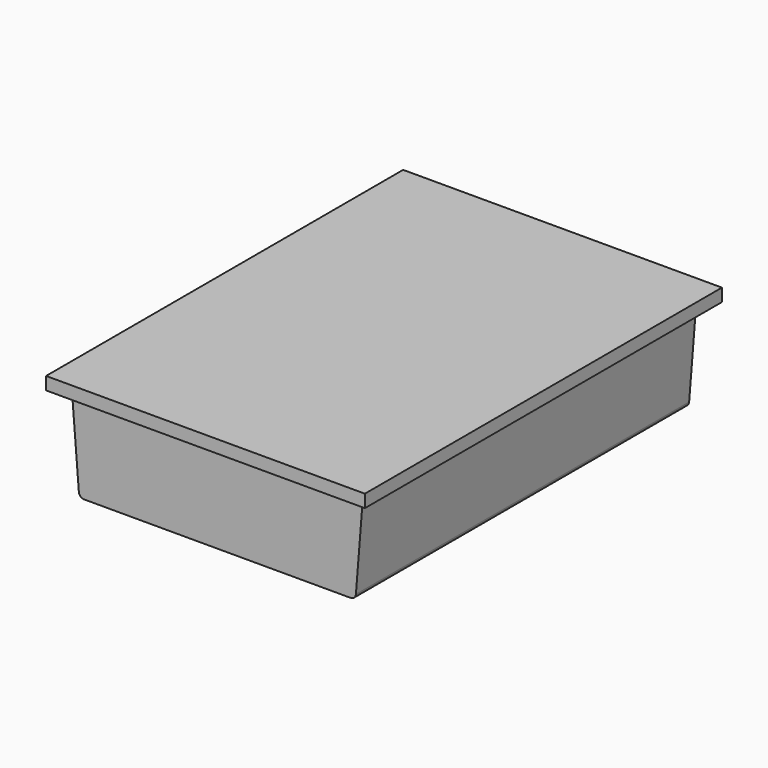
from build123d import *

# Parameters (mm, degrees)
F1_DEPTH = 420
F3_DEPTH = 14


# Not quite as in the source:
# - a pattern or mirror of a feature is missing from the dataset's text; its kind, count and spacing are read off the source's solid


with BuildPart() as f1:
    # F0 (on Front) → F1 (new body)
    with BuildSketch(Plane.XZ):
        with BuildLine():
            Line((150, 0), (0, 0))
            Line((0, 0), (-150, 0))
            Line((-150, 0), (-150, -12))
            Line((-150, -12), (-141.6180664814, -12))
            ThreePointArc((-141.6180664814, -12), (-138.2256023722, -13.3269648425), (-136.633810504, -16.6035250927))
            Line((-136.633810504, -16.6035250927), (-130.366189496, -95.3964749073))
            ThreePointArc((-130.366189496, -95.3964749073), (-128.7743976278, -98.6730351575), (-125.3819335186, -100))
            Line((-125.3819335186, -100), (0, -100))
            Line((0, -100), (125.3819335186, -100))
            ThreePointArc((125.3819335186, -100), (128.7743976278, -98.6730351575), (130.366189496, -95.3964749073))
            Line((130.366189496, -95.3964749073), (136.633810504, -16.6035250927))
            ThreePointArc((136.633810504, -16.6035250927), (138.2256023722, -13.3269648425), (141.6180664814, -12))
            Line((141.6180664814, -12), (150, -12))
            Line((150, -12), (150, 0))
        make_face()
    extrude(amount=F1_DEPTH)

    # F2 (on face) → F3 (cut)
    with BuildSketch(Plane.XZ.offset(420)):
        with BuildLine():
            Line((141.6180664814, -12), (-141.6180664814, -12))
            ThreePointArc((-141.6180664814, -12), (-138.2256023722, -13.3269648425), (-136.633810504, -16.6035250927))
            Line((-136.633810504, -16.6035250927), (-130.366189496, -95.3964749073))
            ThreePointArc((-130.366189496, -95.3964749073), (-128.7743976278, -98.6730351575), (-125.3819335186, -100))
            Line((-125.3819335186, -100), (125.3819335186, -100))
            ThreePointArc((125.3819335186, -100), (128.7743976278, -98.6730351575), (130.366189496, -95.3964749073))
            Line((130.366189496, -95.3964749073), (136.633810504, -16.6035250927))
            ThreePointArc((136.633810504, -16.6035250927), (138.2256023722, -13.3269648425), (141.6180664814, -12))
        make_face()
    f3 = extrude(amount=-F3_DEPTH, mode=Mode.SUBTRACT)

    # F3_copies: F3 across plane
    add(f3.mirror(Plane.ZX.offset(-210)), mode=Mode.SUBTRACT)


solid = f1.part
